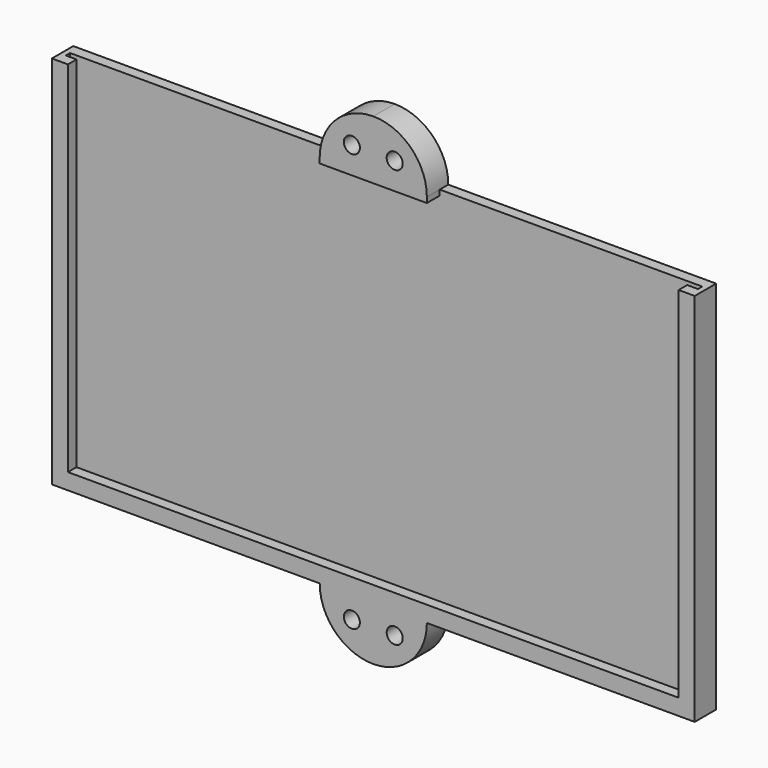
from build123d import *

# Parameters (mm, degrees)
F0_W      = 120
F0_H      = 70
F1_DEPTH  = 2
F3_DEPTH  = 1
F5_DEPTH  = 2
F6_W      = 20
F6_H      = 1
F7_DEPTH  = 3
F9_DEPTH  = 5
F11_DEPTH = 5
F12_R     = 1.5
F13_DEPTH = 5.001


# Not quite as in the source:
# - a feature names something its author has since deleted; it is built from what else it names


with BuildPart() as f1:
    # F0 (on Front) → F1 (new body)
    with BuildSketch(Plane.XZ):
        Rectangle(F0_W, F0_H)
    extrude(amount=F1_DEPTH)

    # F2 (on face) → F3 (join)
    with BuildSketch(Plane.XZ.offset(2)):
        Polygon((-59, -34), (-59, 35), (-60, 35), (-60, -35), (60, -35), (60, 35), (59, 35), (59, -34), align=None)
    extrude(amount=F3_DEPTH)

    # F4 (on face) → F5 (join)
    with BuildSketch(Plane.XZ.offset(3)):
        Polygon((-57, 35), (-60, 35), (-60, -35), (60, -35), (60, 35), (57, 35), (57, -32), (-57, -32), align=None)
    extrude(amount=F5_DEPTH)

    # F6 (on face) → F7 (join)
    with BuildSketch(Plane.XZ.offset(2)):
        with Locations((0, 34.5)):
            Rectangle(F6_W, F6_H)
    extrude(amount=F7_DEPTH)

    # F8 (on face) → F9 (join)
    with BuildSketch(Plane.XZ.offset(5)):
        with BuildLine():
            ThreePointArc((0, 45), (-7.0710678119, 42.0710678119), (-10, 35))
            Line((-10, 35), (10, 35))
            ThreePointArc((10, 35), (7.0710678119, 42.0710678119), (0, 45))
        make_face()
    extrude(amount=-F9_DEPTH)

    # F10 (on face) → F11 (join)
    with BuildSketch(Plane.XZ.offset(5)):
        with BuildLine():
            Line((10, -35), (-10, -35))
            ThreePointArc((-10, -35), (-7.0710678119, -42.0710678119), (0, -45))
            ThreePointArc((0, -45), (7.0710678119, -42.0710678119), (10, -35))
        make_face()
    extrude(amount=-F11_DEPTH)

    # F12 (on face) → F13 (cut, through all)
    with BuildSketch(Plane.XZ.offset(5)):
        with Locations((-4, -39)):
            Circle(F12_R)
        with Locations((4, -39)):
            Circle(F12_R)
        with Locations((-4, 39)):
            Circle(F12_R)
        with Locations((4, 39)):
            Circle(F12_R)
    extrude(amount=-F13_DEPTH, mode=Mode.SUBTRACT)


solid = f1.part
